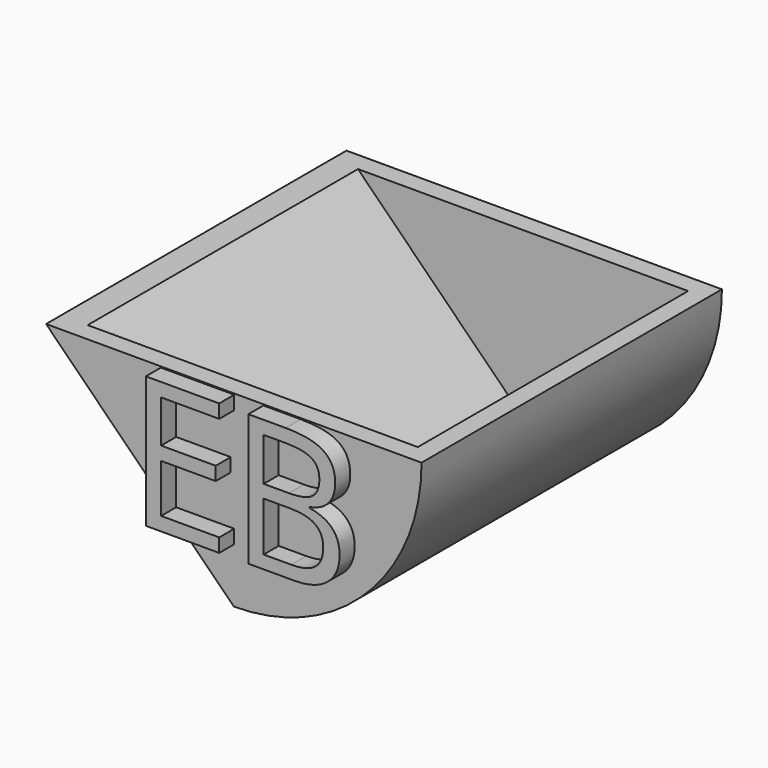
from build123d import *

# Parameters (mm, degrees)
F1_DEPTH     = 50.8
F2_T         = -2.54
F3_TEXT_SIZE = 24.9451558919
F4_DEPTH     = 2.54


# Not quite as in the source:
# - Text() gives the source's letters only with a copy of the font that has no kerning and outlines rounded to 1/6400 em; it was checked with that copy


with BuildPart() as f1:
    # F0 (on Front) → F1 (new body)
    with BuildSketch(Plane.XZ):
        with BuildLine():
            Line((0, 1.6014038861), (-50.8, 1.6014038861))
            Line((-50.8, 1.6014038861), (-25.4, -23.7985961139))
            ThreePointArc((-25.4, -23.7985961139), (-7.4394877579, -16.3591083561), (0, 1.6014038861))
        make_face()
    extrude(amount=F1_DEPTH)

    # F2
    f2_openings = [f1.faces().sort_by_distance(p)[0] for p in [
        (-25.4, -25.4, 1.601404),
    ]]
    offset(amount=F2_T, openings=f2_openings)

    # F3 (on face) → F4 (join)
    with BuildSketch(Plane.XZ.offset(50.8)):
        with Locations((-37.7166707216, -16.3591083561)):
            Text('EB', F3_TEXT_SIZE, font='Open Sans', text_align=(TextAlign.LEFT, TextAlign.BOTTOM))
    extrude(amount=F4_DEPTH)


solid = f1.part
